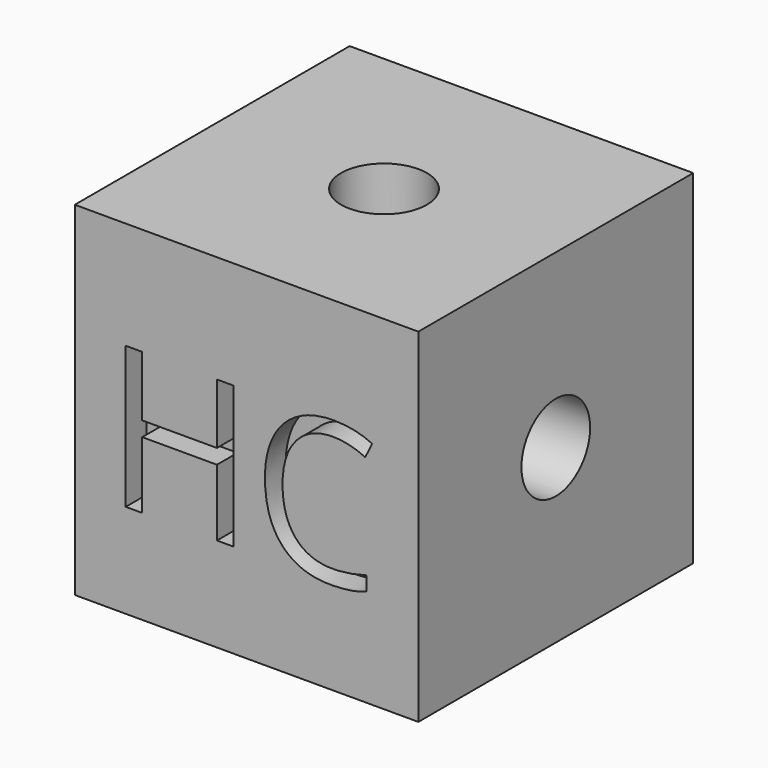
from build123d import *

# Parameters (mm, degrees)
F0_W         = 40
F0_H         = 40
F1_DEPTH     = 40
F2_TEXT_SIZE = 23.1229027526
F3_DEPTH     = 3
F4_R         = 5
F5_DEPTH     = 10
F6_R         = 5
F7_DEPTH     = 10
F8_R         = 5
F9_DEPTH     = 10
F10_R        = 5
F11_DEPTH    = 10
F12_R        = 5
F13_DEPTH    = 10


# Not quite as in the source:
# - Text() gives the source's letters only with a copy of the font that has no kerning and outlines rounded to 1/6400 em; it was checked with that copy


with BuildPart() as f1:
    # F0 (on Front) → F1 (new body)
    with BuildSketch(Plane.XZ):
        with Locations((-20, 20)):
            Rectangle(F0_W, F0_H)
    extrude(amount=F1_DEPTH)

    # F2 (on face) → F3 (cut)
    with BuildSketch(Plane.XZ.offset(40)):
        with Locations((-36.3359926268, 10.9668634832)):
            Text('HC', F2_TEXT_SIZE, font='Open Sans', text_align=(TextAlign.LEFT, TextAlign.BOTTOM))
    extrude(amount=-F3_DEPTH, mode=Mode.SUBTRACT)

    # F4 (on face) → F5 (cut)
    with BuildSketch(Plane.YZ):
        with Locations((-20, 20)):
            Circle(F4_R)
    extrude(amount=-F5_DEPTH, mode=Mode.SUBTRACT)

    # F6 (on face) → F7 (cut)
    with BuildSketch(Plane(origin=(-40, 0, 0), x_dir=(0, -1, 0), z_dir=(-1, 0, 0))):
        with Locations((20, 20)):
            Circle(F6_R)
    extrude(amount=-F7_DEPTH, mode=Mode.SUBTRACT)

    # F8 (on face) → F9 (cut)
    with BuildSketch(Plane.XY.offset(40)):
        with Locations((-20, -20)):
            Circle(F8_R)
    extrude(amount=-F9_DEPTH, mode=Mode.SUBTRACT)

    # F10 (on face) → F11 (cut)
    with BuildSketch(Plane(origin=(0, 0, 0), x_dir=(1, 0, 0), z_dir=(0, 0, -1))):
        with Locations((-20, 20)):
            Circle(F10_R)
    extrude(amount=-F11_DEPTH, mode=Mode.SUBTRACT)

    # F12 (on face) → F13 (cut)
    with BuildSketch(Plane(origin=(0, 0, 0), x_dir=(-1, 0, 0), z_dir=(0, 1, 0))):
        with Locations((20, 20)):
            Circle(F12_R)
    extrude(amount=-F13_DEPTH, mode=Mode.SUBTRACT)


solid = f1.part
